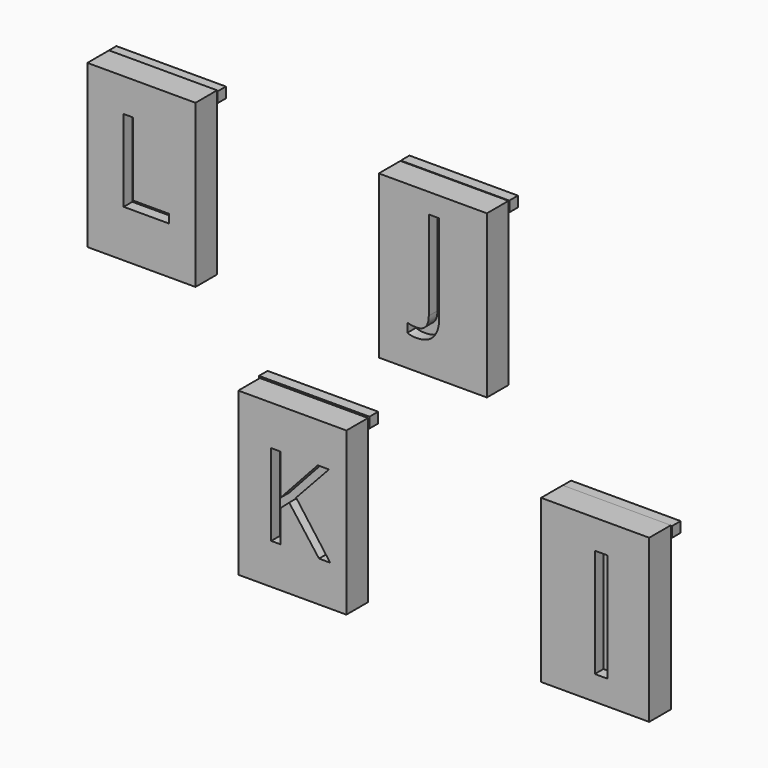
from build123d import *

# Parameters (mm, degrees)
F0_W           = 25.4
F0_H           = 38.1
F1_DEPTH       = 6.35
F2_R           = 3.81
F3_DEPTH       = 2.54
F5_TEXT_SIZE   = 35.7440258894
F5_TEXT_SIZE_2 = 29.3738053491
F5_TEXT_SIZE_3 = 26.8964970019
F6_DEPTH       = 25.4
F7_W           = 25.730624795
F7_H           = 2.4505369365
F8_DEPTH       = 2.54
F7_W_2         = 25.4855751991
F7_W_3         = 25.7306285203
F7_W_4         = 25.9756827727
F7_H_2         = 2.4505350739


# Not quite as in the source:
# - Text() gives the source's letters only with a copy of the font that has no kerning and outlines rounded to 1/6400 em; it was checked with that copy


with BuildPart() as f1:
    # F0 (on Front) → F1 (new body)
    with BuildSketch(Plane.XZ):
        with Locations((-46.0602159804, 19.2970331914)):
            Rectangle(F0_W, F0_H)
    extrude(amount=F1_DEPTH)

    # F2 (on Front) → F3, piece 3 (join)
    with BuildSketch(Plane.XZ):
        with Locations((-40.9802159804, 28.1870331914)):
            Circle(F2_R)
        with Locations((-40.9802159804, 18.0270331914)):
            Circle(F2_R)
        with Locations((-40.9802159804, 7.8670331914)):
            Circle(F2_R)
    extrude(amount=-F3_DEPTH)


with BuildPart() as f1b:
    # F0 (on Front) → F1, piece 2 (new body)
    with BuildSketch(Plane.XZ):
        with Locations((-10.603061258, -36.9614025138)):
            Rectangle(F0_W, F0_H)
    extrude(amount=F1_DEPTH)

    # F2 (on Front) → F3, piece 2 (join)
    with BuildSketch(Plane.XZ):
        with Locations((-5.523061258, -28.0714025138)):
            Circle(F2_R)
        with Locations((-5.523061258, -48.3914025138)):
            Circle(F2_R)
    extrude(amount=-F3_DEPTH)


with BuildPart() as f1c:
    # F0 (on Front) → F1, piece 3 (new body)
    with BuildSketch(Plane.XZ):
        with Locations((60.5514380593, -36.0065931796)):
            Rectangle(F0_W, F0_H)
    extrude(amount=F1_DEPTH)

    # F2 (on Front) → F3, piece 4 (join)
    with BuildSketch(Plane.XZ):
        with Locations((65.6314380593, -37.2765931796)):
            Circle(F2_R)
        with Locations((55.4714380593, -27.1165931796)):
            Circle(F2_R)
    extrude(amount=-F3_DEPTH)


with BuildPart() as f1d:
    # F0 (on Front) → F1, piece 4 (new body)
    with BuildSketch(Plane.XZ):
        with Locations((22.4085926682, 18.6961098781)):
            Rectangle(F0_W, F0_H)
    extrude(amount=F1_DEPTH)

    # F2 (on Front) → F3 (join)
    with BuildSketch(Plane.XZ):
        with Locations((27.4885926682, 17.4261098781)):
            Circle(F2_R)
        with Locations((17.3285926682, 27.5861098781)):
            Circle(F2_R)
        with Locations((17.3285926682, 17.4261098781)):
            Circle(F2_R)
    extrude(amount=-F3_DEPTH)


with BuildPart() as f6_tool:
    # F5 (on offset) → F6 (new body)
    with BuildSketch(Plane.XZ.offset(3.81)):
        with Locations((56.9497905672, -49.3055284023)):
            Text('I', F5_TEXT_SIZE, font='Open Sans', text_align=(TextAlign.LEFT, TextAlign.BOTTOM))
        with Locations((18.7284704298, 12.1034244075)):
            Text('J', F5_TEXT_SIZE_2, font='Open Sans', text_align=(TextAlign.LEFT, TextAlign.BOTTOM))
        with Locations((-18.2188414037, -46.502626501)):
            Text('K', F5_TEXT_SIZE_3, font='Open Sans', text_align=(TextAlign.LEFT, TextAlign.BOTTOM))
        with Locations((-52.8728477657, 11.3389985636)):
            Text('L', F5_TEXT_SIZE_3, font='Open Sans', text_align=(TextAlign.LEFT, TextAlign.BOTTOM))
    extrude(amount=F6_DEPTH)


with BuildPart() as f1_1:
    add(f1.part)

    # F6: cut by f6_tool
    add(f6_tool.part, mode=Mode.SUBTRACT)

    # F7 (on Front) → F8, piece 3 (join)
    with BuildSketch(Plane.XZ):
        with Locations((-46.1926031858, 36.8805658072)):
            Rectangle(F7_W_3, F7_H)
    extrude(amount=-F8_DEPTH)


with BuildPart() as f1b_1:
    add(f1b.part)

    # F6: cut by f6_tool
    add(f6_tool.part, mode=Mode.SUBTRACT)

    # F7 (on Front) → F8, piece 4 (join)
    with BuildSketch(Plane.XZ):
        with Locations((-10.5373053811, -18.7466004863)):
            Rectangle(F7_W_4, F7_H_2)
    extrude(amount=-F8_DEPTH)


with BuildPart() as f1c_1:
    add(f1c.part)

    # F6: cut by f6_tool
    add(f6_tool.part, mode=Mode.SUBTRACT)

    # F7 (on Front) → F8 (join)
    with BuildSketch(Plane.XZ):
        with Locations((60.6507658958, -18.2564929128)):
            Rectangle(F7_W, F7_H)
    extrude(amount=-F8_DEPTH)


with BuildPart() as f1d_1:
    add(f1d.part)

    # F6: cut by f6_tool
    add(f6_tool.part, mode=Mode.SUBTRACT)

    # F7 (on Front) → F8, piece 2 (join)
    with BuildSketch(Plane.XZ):
        with Locations((22.5449316204, 36.6355124861)):
            Rectangle(F7_W_2, F7_H)
    extrude(amount=-F8_DEPTH)


solid = Compound([f1_1.part, f1b_1.part, f1c_1.part, f1d_1.part])
